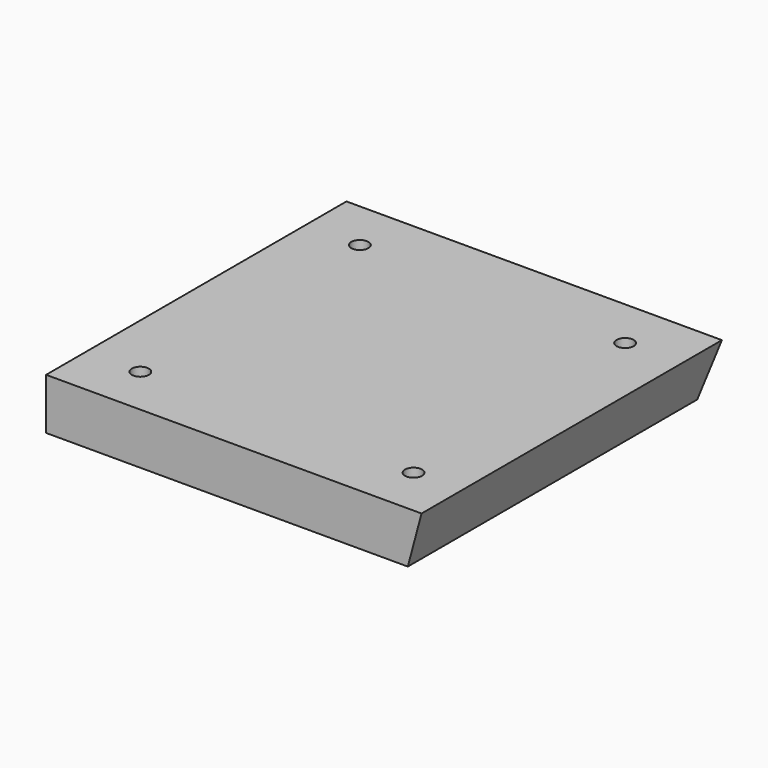
from build123d import *

# Parameters (mm, degrees)
F0_W     = 139.7
F0_H     = 139.7
F0_R     = 3.175
F1_DEPTH = 19.05
F2_SIZE2 = 5.104422
F2_SIZE  = 19.04999


# Not quite as in the source:
# - a fillet or chamfer is up to 0.001 mm smaller than in the source, because OpenCascade refuses the exact size


with BuildPart() as f1:
    # F0 (on Top) → F1 (new body)
    with BuildSketch(Plane.XY):
        with Locations((-3.4590801224, 34.0288509236)):
            Rectangle(F0_W, F0_H)
        with Locations((-53.1284622848, -17.2076094896)):
            Circle(F0_R, mode=Mode.SUBTRACT)
        with Locations((48.5374927521, -17.2076094896)):
            Circle(F0_R, mode=Mode.SUBTRACT)
        with Locations((-53.1284622848, 84.8837196827)):
            Circle(F0_R, mode=Mode.SUBTRACT)
        with Locations((45.559823513, 84.8837196827)):
            Circle(F0_R, mode=Mode.SUBTRACT)
    extrude(amount=F1_DEPTH)

    # F2 (size 19.05 and 5.1044321158 in the source; OpenCascade refuses exactly that, so slightly less here)
    f2_edges = [f1.edges().sort_by_distance(p)[0] for p in [
        (66.39092, 34.028851, 0),
        (-3.45908, 103.878851, 0),
    ]]
    chamfer(f2_edges, length=F2_SIZE, length2=F2_SIZE2)


solid = f1.part
